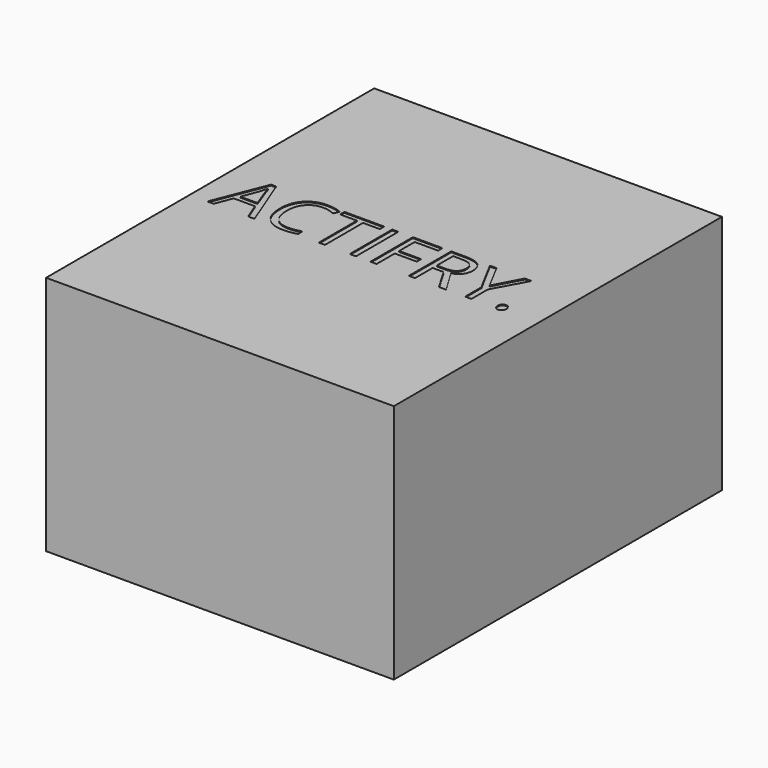
from build123d import *

# Parameters (mm, degrees)
F0_W         = 390
F0_H         = 460
F1_DEPTH     = 270
F2_TEXT_SIZE = 83.3333333333
F3_DEPTH     = 1


# Not quite as in the source:
# - Text() gives the source's letters only with a copy of the font that has no kerning and outlines rounded to 1/6400 em; it was checked with that copy


with BuildPart() as f1:
    # F0 (on Top) → F1 (new body)
    with BuildSketch(Plane.XY):
        Rectangle(F0_W, F0_H)
    extrude(amount=F1_DEPTH)

    # F2 (on face) → F3 (cut)
    with BuildSketch(Plane.XY.offset(270)):
        with Locations((-175, -28.7422219877)):
            Text('ACTIFRY.', F2_TEXT_SIZE, font='Open Sans', text_align=(TextAlign.LEFT, TextAlign.BOTTOM))
    extrude(amount=-F3_DEPTH, mode=Mode.SUBTRACT)


solid = f1.part
